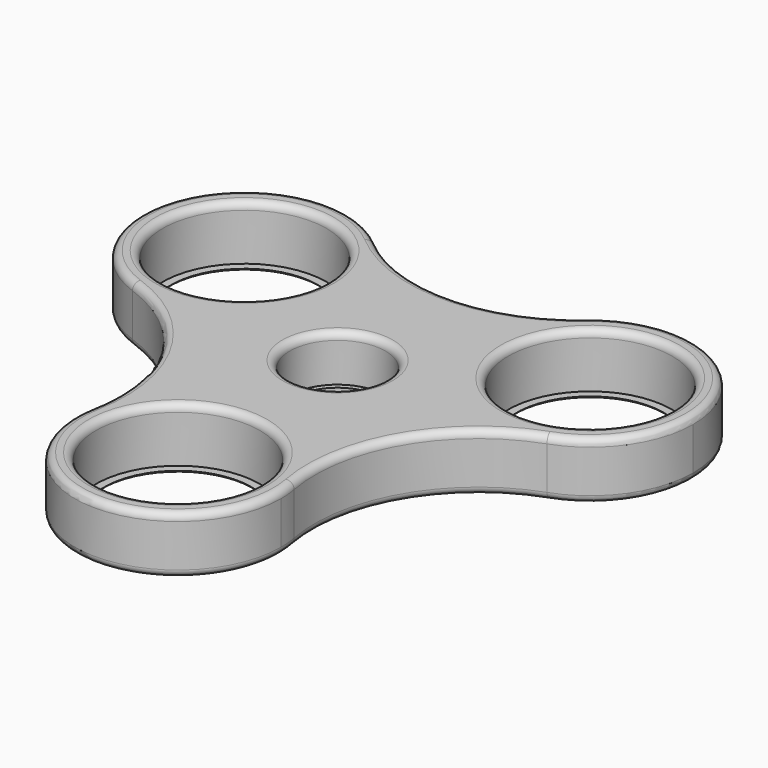
from build123d import *

# Parameters (mm, degrees)
F0_R         = 6.5
F0_R_2       = 11.15
F1_DEPTH     = 7.8
F2_R         = 11.15
F2_R_2       = 10
F3_DEPTH     = 0.4
F4_R         = 6.5
F4_R_2       = 5.8
F5_DEPTH     = 1.5
F6_T10_ANGLE = 80.8915948213
F6_T12_ANGLE = 200.8915947618
F6_T14_ANGLE = 80.8915945525
F6_T16_ANGLE = 200.8915947547
F6_T18_ANGLE = 80.8915942666
F6_T20_ANGLE = 200.8915950895
F6_T22_ANGLE = 80.8915948213
F6_T24_ANGLE = 200.8915947618
F6_T26_ANGLE = 80.8915945525
F6_T28_ANGLE = 200.8915947547
F6_T30_ANGLE = 80.8915942666
F6_T32_ANGLE = 200.8915950895


# Not quite as in the source:
# - a fillet or chamfer that OpenCascade refuses, or shapes differently, is made with other operations: its cross-section is extruded or revolved along the edge and cut away or added


with BuildPart() as f1:
    # F0 (on Top) → F1 (new body)
    with BuildSketch(Plane.XY):
        with BuildLine():
            ThreePointArc((-14.4178023884, 24.2220115243), (-10.7887694034, 19.434980828), (-9.5, 13.567731326))
            ThreePointArc((-9.5, 13.567731326), (-15.4253761081, 2.1309289317), (-28.1857784292, 0.3751773461))
            ThreePointArc((-28.1857784292, 0.3751773461), (-17.4686665105, -7.7494316525), (-13.3996429494, -20.567731326))
            ThreePointArc((-13.3996429494, -20.567731326), (-13.4919177982, -22.5908599334), (-13.7679761122, -24.5971888737))
            ThreePointArc((-13.7679761122, -24.5971888737), (-1.54e-08, -13.1354626519), (13.7679761066, -24.5971888434))
            ThreePointArc((13.7679761066, -24.5971888434), (16.3771898334, -9.4553750199), (28.1857783538, 0.3751773193))
            ThreePointArc((28.1857783538, 0.3751773193), (11.3756443069, 6.5677313954), (14.4178023884, 24.2220115243))
            ThreePointArc((14.4178023884, 24.2220115243), (0, 18.9107499483), (-14.4178023884, 24.2220115243))
        make_face()
        Circle(F0_R, mode=Mode.SUBTRACT)
        with BuildLine():
            ThreePointArc((-28.1857784292, 0.3751773461), (-15.4253761081, 2.1309289317), (-9.5, 13.567731326))
            ThreePointArc((-9.5, 13.567731326), (-10.7887694034, 19.434980828), (-14.4178023884, 24.2220115243))
            ThreePointArc((-14.4178023884, 24.2220115243), (-35.6243556731, 20.5677312911), (-28.1857784292, 0.3751773461))
        make_face()
        with Locations((-23.5, 13.567731326)):
            Circle(F0_R_2, mode=Mode.SUBTRACT)
        with BuildLine():
            ThreePointArc((37.5, 13.567731326), (29.367249502, 26.2789619226), (14.4178023884, 24.2220115243))
            ThreePointArc((14.4178023884, 24.2220115243), (11.3756443069, 6.5677313954), (28.1857783538, 0.3751773193))
            ThreePointArc((28.1857783538, 0.3751773193), (34.9368023711, 5.4931074014), (37.5, 13.567731326))
        make_face()
        with Locations((23.5, 13.567731326)):
            Circle(F0_R_2, mode=Mode.SUBTRACT)
        with BuildLine():
            ThreePointArc((13.7679761066, -24.5971888434), (-1.54e-08, -13.1354626519), (-13.7679761122, -24.5971888737))
            ThreePointArc((-13.7679761122, -24.5971888737), (-1.2744281911, -41.0773360119), (14, -27.1354626519))
            ThreePointArc((14, -27.1354626519), (13.9418733586, -25.8610344454), (13.7679761066, -24.5971888434))
        make_face()
        with Locations((0, -27.1354626519)):
            Circle(F0_R_2, mode=Mode.SUBTRACT)
    extrude(amount=F1_DEPTH)

    # F2 (on face) → F3 (join)
    with BuildSketch(Plane(origin=(0, 0, 0), x_dir=(1, 0, 0), z_dir=(0, 0, -1))):
        with Locations((0, 27.1354626519)):
            Circle(F2_R)
        with Locations((0, 27.1354626519)):
            Circle(F2_R_2, mode=Mode.SUBTRACT)
        with Locations((23.5, -13.567731326)):
            Circle(F2_R)
        with Locations((23.5, -13.567731326)):
            Circle(F2_R_2, mode=Mode.SUBTRACT)
        with Locations((-23.5, -13.567731326)):
            Circle(F2_R)
        with Locations((-23.5, -13.567731326)):
            Circle(F2_R_2, mode=Mode.SUBTRACT)
    extrude(amount=-F3_DEPTH)

    # F4 (on face) → F5 (join)
    with BuildSketch(Plane(origin=(0, 0, 0), x_dir=(1, 0, 0), z_dir=(0, 0, -1))):
        Circle(F4_R)
        Circle(F4_R_2, mode=Mode.SUBTRACT)
    extrude(amount=-F5_DEPTH)

    # F6: fillet of radius 1 on 20 edges, made by hand

    # F6_s1 → F6_t2 (revolve, cut)
    with BuildSketch(Plane.XZ.offset(-13.567731326)):
        with BuildLine():
            ThreePointArc((-11.35, 7.8), (-12.0571067812, 7.5071067812), (-12.35, 6.8))
            Line((-12.35, 6.8), (-12.35, 7.8))
            Line((-12.35, 7.8), (-11.35, 7.8))
        make_face()
    revolve(axis=Axis((-23.5, 13.567731326, 7.8), (0, 0, 1)), mode=Mode.SUBTRACT)

    # F6_s3 → F6_t4 (revolve, cut)
    with BuildSketch(Plane.XZ.offset(27.1354626519)):
        with BuildLine():
            ThreePointArc((12.15, 7.8), (11.4428932188, 7.5071067812), (11.15, 6.8))
            Line((11.15, 6.8), (11.15, 7.8))
            Line((11.15, 7.8), (12.15, 7.8))
        make_face()
    revolve(axis=Axis((0, -27.1354626519, 7.8), (0, 0, 1)), mode=Mode.SUBTRACT)

    # F6_s5 → F6_t6 (revolve, cut)
    with BuildSketch(Plane.XZ):
        with BuildLine():
            ThreePointArc((7.5, 7.8), (6.7928932188, 7.5071067812), (6.5, 6.8))
            Line((6.5, 6.8), (6.5, 7.8))
            Line((6.5, 7.8), (7.5, 7.8))
        make_face()
    revolve(axis=Axis((0, 0, 7.8), (0, 0, 1)), mode=Mode.SUBTRACT)

    # F6_s7 → F6_t8 (revolve, cut)
    with BuildSketch(Plane.XZ.offset(-13.567731326)):
        with BuildLine():
            ThreePointArc((35.65, 7.8), (34.9428932188, 7.5071067812), (34.65, 6.8))
            Line((34.65, 6.8), (34.65, 7.8))
            Line((34.65, 7.8), (35.65, 7.8))
        make_face()
    revolve(axis=Axis((23.5, 13.567731326, 7.8), (0, 0, 1)), mode=Mode.SUBTRACT)

    # F6_s9 → F6_t10 (revolve, cut)
    with BuildSketch(Plane(origin=(20.3083844645, 17.3117994564, 0), x_dir=(0, 0, 1), z_dir=(0.761020012, 0.6487284034, 0))):
        with BuildLine():
            ThreePointArc((6.8, -9.0801975759), (7.5071067812, -8.7873043571), (7.8, -8.0801975759))
            Line((7.8, -8.0801975759), (7.8, -9.0801975759))
            Line((7.8, -9.0801975759), (6.8, -9.0801975759))
        make_face()
    revolve(axis=Axis((0, 41.1354626519, 7.8), (0, 0, -1)), revolution_arc=F6_T10_ANGLE, mode=Mode.SUBTRACT)

    # F6_s11 → F6_t12 (revolve, cut)
    with BuildSketch(Plane(origin=(-20.3083844997, 17.3117993675, 0), x_dir=(0, 0, 1), z_dir=(0.7610200142, -0.6487284008, 0))):
        with BuildLine():
            ThreePointArc((6.8, -9.0801976664), (7.5071067812, -8.7873044476), (7.8, -8.0801976664))
            Line((7.8, -8.0801976664), (7.8, -9.0801976664))
            Line((7.8, -9.0801976664), (6.8, -9.0801976664))
        make_face()
    revolve(axis=Axis((-23.5, 13.567731326, 7.8), (0, 0, 1)), revolution_arc=F6_T12_ANGLE, mode=Mode.SUBTRACT)

    # F6_s13 → F6_t14 (revolve, cut)
    with BuildSketch(Plane(origin=(-25.1466502077, 8.9316771809, 0), x_dir=(0, 0, 1), z_dir=(-0.9423252823, 0.3346984649, 0))):
        with BuildLine():
            ThreePointArc((7.8, -8.0801976725), (7.5071067812, -8.7873044537), (6.8, -9.0801976725))
            Line((6.8, -9.0801976725), (7.8, -9.0801976725))
            Line((7.8, -9.0801976725), (7.8, -8.0801976725))
        make_face()
    revolve(axis=Axis((-35.624355653, -20.567731326, 7.8), (0, 0, -1)), revolution_arc=F6_T14_ANGLE, mode=Mode.SUBTRACT)

    # F6_s15 → F6_t16 (revolve, cut)
    with BuildSketch(Plane(origin=(-4.8382658309, -26.2434765539, 0), x_dir=(0, 0, 1), z_dir=(0.1813052699, 0.9834268652, 0))):
        with BuildLine():
            ThreePointArc((7.8, -8.0801976209), (7.5071067812, -8.787304402), (6.8, -9.0801976209))
            Line((6.8, -9.0801976209), (7.8, -9.0801976209))
            Line((7.8, -9.0801976209), (7.8, -8.0801976209))
        make_face()
    revolve(axis=Axis((0, -27.1354626519, 7.8), (0, 0, 1)), revolution_arc=F6_T16_ANGLE, mode=Mode.SUBTRACT)

    # F6_s17 → F6_t18 (revolve, cut)
    with BuildSketch(Plane(origin=(4.8382658036, -26.2434765203, 0), x_dir=(0, 0, 1), z_dir=(0.1813052691, -0.9834268653, 0))):
        with BuildLine():
            ThreePointArc((7.8, -8.0801976417), (7.5071067812, -8.7873044229), (6.8, -9.0801976417))
            Line((6.8, -9.0801976417), (7.8, -9.0801976417))
            Line((7.8, -9.0801976417), (7.8, -8.0801976417))
        make_face()
    revolve(axis=Axis((35.624355653, -20.567731326, 7.8), (0, 0, -1)), revolution_arc=F6_T18_ANGLE, mode=Mode.SUBTRACT)

    # F6_s19 → F6_t20 (revolve, cut)
    with BuildSketch(Plane(origin=(25.1466503366, 8.9316768958, 0), x_dir=(0, 0, 1), z_dir=(-0.9423252862, -0.3346984538, 0))):
        with BuildLine():
            ThreePointArc((6.8, -9.0801973606), (7.5071067812, -8.7873041418), (7.8, -8.0801973606))
            Line((7.8, -8.0801973606), (7.8, -9.0801973606))
            Line((7.8, -9.0801973606), (6.8, -9.0801973606))
        make_face()
    revolve(axis=Axis((23.5, 13.567731326, 7.8), (0, 0, 1)), revolution_arc=F6_T20_ANGLE, mode=Mode.SUBTRACT)

    # F6_s21 → F6_t22 (revolve, cut)
    with BuildSketch(Plane(origin=(20.3083844645, 17.3117994564, 0), x_dir=(0, 0, 1), z_dir=(0.761020012, 0.6487284034, 0))):
        with BuildLine():
            ThreePointArc((1, -9.0801975759), (0.2928932188, -8.7873043571), (0, -8.0801975759))
            Line((0, -8.0801975759), (0, -9.0801975759))
            Line((0, -9.0801975759), (1, -9.0801975759))
        make_face()
    revolve(axis=Axis((0, 41.1354626519, 0), (0, 0, -1)), revolution_arc=F6_T22_ANGLE, mode=Mode.SUBTRACT)

    # F6_s23 → F6_t24 (revolve, cut)
    with BuildSketch(Plane(origin=(-20.3083844997, 17.3117993675, 0), x_dir=(0, 0, 1), z_dir=(0.7610200142, -0.6487284008, 0))):
        with BuildLine():
            ThreePointArc((1, -9.0801976664), (0.2928932188, -8.7873044476), (0, -8.0801976664))
            Line((0, -8.0801976664), (0, -9.0801976664))
            Line((0, -9.0801976664), (1, -9.0801976664))
        make_face()
    revolve(axis=Axis((-23.5, 13.567731326, 0), (0, 0, 1)), revolution_arc=F6_T24_ANGLE, mode=Mode.SUBTRACT)

    # F6_s25 → F6_t26 (revolve, cut)
    with BuildSketch(Plane(origin=(-25.1466502077, 8.9316771809, 0), x_dir=(0, 0, 1), z_dir=(-0.9423252823, 0.3346984649, 0))):
        with BuildLine():
            ThreePointArc((0, -8.0801976725), (0.2928932188, -8.7873044537), (1, -9.0801976725))
            Line((1, -9.0801976725), (0, -9.0801976725))
            Line((0, -9.0801976725), (0, -8.0801976725))
        make_face()
    revolve(axis=Axis((-35.624355653, -20.567731326, 0), (0, 0, -1)), revolution_arc=F6_T26_ANGLE, mode=Mode.SUBTRACT)

    # F6_s27 → F6_t28 (revolve, cut)
    with BuildSketch(Plane(origin=(-4.8382658309, -26.2434765539, 0), x_dir=(0, 0, 1), z_dir=(0.1813052699, 0.9834268652, 0))):
        with BuildLine():
            ThreePointArc((0, -8.0801976209), (0.2928932188, -8.787304402), (1, -9.0801976209))
            Line((1, -9.0801976209), (0, -9.0801976209))
            Line((0, -9.0801976209), (0, -8.0801976209))
        make_face()
    revolve(axis=Axis((0, -27.1354626519, 0), (0, 0, 1)), revolution_arc=F6_T28_ANGLE, mode=Mode.SUBTRACT)

    # F6_s29 → F6_t30 (revolve, cut)
    with BuildSketch(Plane(origin=(4.8382658036, -26.2434765203, 0), x_dir=(0, 0, 1), z_dir=(0.1813052691, -0.9834268653, 0))):
        with BuildLine():
            ThreePointArc((0, -8.0801976417), (0.2928932188, -8.7873044229), (1, -9.0801976417))
            Line((1, -9.0801976417), (0, -9.0801976417))
            Line((0, -9.0801976417), (0, -8.0801976417))
        make_face()
    revolve(axis=Axis((35.624355653, -20.567731326, 0), (0, 0, -1)), revolution_arc=F6_T30_ANGLE, mode=Mode.SUBTRACT)

    # F6_s31 → F6_t32 (revolve, cut)
    with BuildSketch(Plane(origin=(25.1466503366, 8.9316768958, 0), x_dir=(0, 0, 1), z_dir=(-0.9423252862, -0.3346984538, 0))):
        with BuildLine():
            ThreePointArc((1, -9.0801973606), (0.2928932188, -8.7873041418), (0, -8.0801973606))
            Line((0, -8.0801973606), (0, -9.0801973606))
            Line((0, -9.0801973606), (1, -9.0801973606))
        make_face()
    revolve(axis=Axis((23.5, 13.567731326, 0), (0, 0, 1)), revolution_arc=F6_T32_ANGLE, mode=Mode.SUBTRACT)

    # F6_s33 → F6_t34 (revolve, cut)
    with BuildSketch(Plane.XZ.offset(-13.567731326)):
        with BuildLine():
            ThreePointArc((-12.7, 0), (-13.1472135955, 0.105572809), (-13.5, 0.4))
            Line((-13.5, 0.4), (-13.5, 0))
            Line((-13.5, 0), (-12.7, 0))
        make_face()
    revolve(axis=Axis((-23.5, 13.567731326, 0), (0, 0, -1)), mode=Mode.SUBTRACT)

    # F6_s35 → F6_t36 (revolve, cut)
    with BuildSketch(Plane.XZ.offset(-13.567731326)):
        with BuildLine():
            ThreePointArc((34.3, 0), (33.8527864045, 0.105572809), (33.5, 0.4))
            Line((33.5, 0.4), (33.5, 0))
            Line((33.5, 0), (34.3, 0))
        make_face()
    revolve(axis=Axis((23.5, 13.567731326, 0), (0, 0, -1)), mode=Mode.SUBTRACT)

    # F6_s37 → F6_t38 (revolve, cut)
    with BuildSketch(Plane.XZ.offset(27.1354626519)):
        with BuildLine():
            ThreePointArc((10.8, 0), (10.3527864045, 0.105572809), (10, 0.4))
            Line((10, 0.4), (10, 0))
            Line((10, 0), (10.8, 0))
        make_face()
    revolve(axis=Axis((0, -27.1354626519, 0), (0, 0, -1)), mode=Mode.SUBTRACT)

    # F6_s39 → F6_t40 (revolve, cut)
    with BuildSketch(Plane.XZ):
        with BuildLine():
            ThreePointArc((6.8, 0), (6.0928932188, 0.2928932188), (5.8, 1))
            Line((5.8, 1), (5.8, 0))
            Line((5.8, 0), (6.8, 0))
        make_face()
    revolve(axis=Axis((0, 0, 0), (0, 0, -1)), mode=Mode.SUBTRACT)


solid = f1.part
